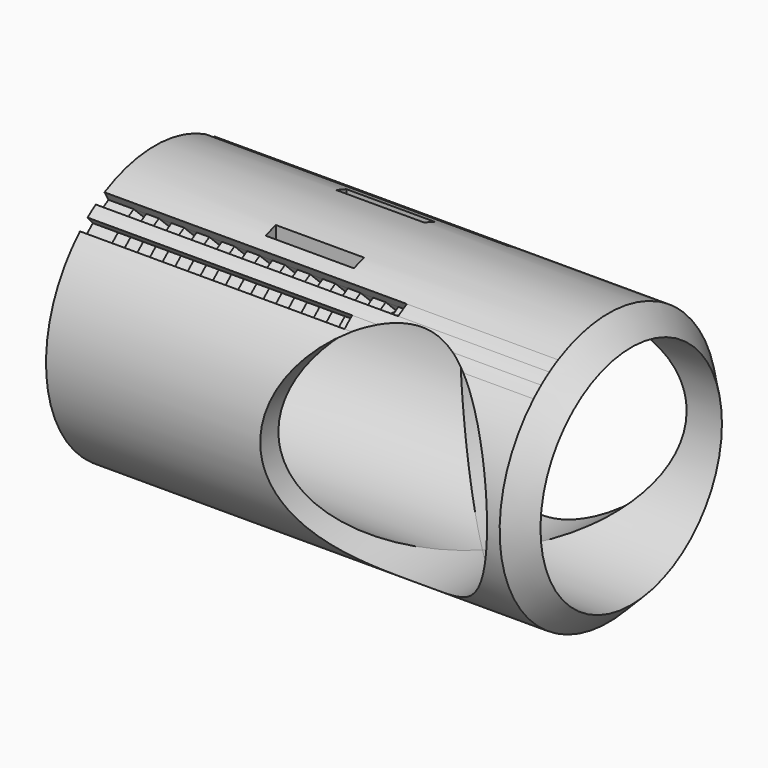
from build123d import *

# Parameters (mm, degrees)
F0_R      = 57.15
F1_DEPTH  = 241.3
F3_DEPTH  = 133.35
F4_DEPTH  = 152.4
F5_DEPTH  = 76.2
F10_ANGLE = 16.3
F11_W     = 44.45
F11_H     = 6.35
F12_DEPTH = 381


# Not quite as in the source:
# - a fillet or chamfer that OpenCascade refuses, or shapes differently, is made with other operations: its cross-section is extruded or revolved along the edge and cut away or added
# - a pattern or mirror of a feature is missing from the dataset's text; its kind, count and spacing are read off the source's solid


with BuildPart() as f1:
    # F0 (on Right) → F1 (new body)
    with BuildSketch(Plane.YZ):
        with BuildLine():
            ThreePointArc((-47.2070556813, 49.7464601143), (-27.0717243759, -63.0106192583), (68.58, 0))
            ThreePointArc((68.58, 0), (63.0106192583, 27.0717243759), (47.2070556813, 49.7464601143))
            Line((47.2070556813, 49.7464601143), (43.8845844861, 45.9035985298))
            Line((43.8845844861, 45.9035985298), (39.0810075056, 50.0566875238))
            Line((39.0810075056, 50.0566875238), (42.4034787008, 53.8995491082))
            ThreePointArc((42.4034787008, 53.8995491082), (39.8626621435, 55.8048794178), (37.2363602362, 57.5905363438))
            Line((37.2363602362, 57.5905363438), (34.6785672677, 53.2014481548))
            Line((34.6785672677, 53.2014481548), (29.1922070315, 56.3986893654))
            Line((29.1922070315, 56.3986893654), (31.75, 60.7877775544))
            ThreePointArc((31.75, 60.7877775544), (0, 68.58), (-31.75, 60.7877775544))
            Line((-31.75, 60.7877775544), (-29.1922070315, 56.3986893654))
            Line((-29.1922070315, 56.3986893654), (-34.6785672677, 53.2014481548))
            Line((-34.6785672677, 53.2014481548), (-37.2363602362, 57.5905363438))
            ThreePointArc((-37.2363602362, 57.5905363438), (-39.8626621435, 55.8048794178), (-42.4034787008, 53.8995491082))
            Line((-42.4034787008, 53.8995491082), (-39.0810075056, 50.0566875238))
            Line((-39.0810075056, 50.0566875238), (-43.8845844861, 45.9035985298))
            Line((-43.8845844861, 45.9035985298), (-47.2070556813, 49.7464601143))
        make_face()
        Circle(F0_R, mode=Mode.SUBTRACT)
        with BuildLine():
            ThreePointArc((-42.4034787008, 53.8995491082), (-44.853361135, 51.8786313899), (-47.2070556813, 49.7464601143))
            Line((-47.2070556813, 49.7464601143), (-43.8845844861, 45.9035985298))
            Line((-43.8845844861, 45.9035985298), (-39.0810075056, 50.0566875238))
            Line((-39.0810075056, 50.0566875238), (-42.4034787008, 53.8995491082))
        make_face()
        with BuildLine():
            ThreePointArc((-31.75, 60.7877775544), (-34.5302050747, 59.2526905507), (-37.2363602362, 57.5905363438))
            Line((-37.2363602362, 57.5905363438), (-34.6785672677, 53.2014481548))
            Line((-34.6785672677, 53.2014481548), (-29.1922070315, 56.3986893654))
            Line((-29.1922070315, 56.3986893654), (-31.75, 60.7877775544))
        make_face()
        with BuildLine():
            Line((34.6785672677, 53.2014481548), (37.2363602362, 57.5905363438))
            ThreePointArc((37.2363602362, 57.5905363438), (34.5302050747, 59.2526905507), (31.75, 60.7877775544))
            Line((31.75, 60.7877775544), (29.1922070315, 56.3986893654))
            Line((29.1922070315, 56.3986893654), (34.6785672677, 53.2014481548))
        make_face()
        with BuildLine():
            Line((43.8845844861, 45.9035985298), (47.2070556813, 49.7464601143))
            ThreePointArc((47.2070556813, 49.7464601143), (44.853361135, 51.8786313899), (42.4034787008, 53.8995491082))
            Line((42.4034787008, 53.8995491082), (39.0810075056, 50.0566875238))
            Line((39.0810075056, 50.0566875238), (43.8845844861, 45.9035985298))
        make_face()
    extrude(amount=F1_DEPTH)

    # F0 (on Right) → F3 (cut)
    with BuildSketch(Plane.YZ):
        with BuildLine():
            ThreePointArc((-42.4034787008, 53.8995491082), (-44.853361135, 51.8786313899), (-47.2070556813, 49.7464601143))
            Line((-47.2070556813, 49.7464601143), (-43.8845844861, 45.9035985298))
            Line((-43.8845844861, 45.9035985298), (-39.0810075056, 50.0566875238))
            Line((-39.0810075056, 50.0566875238), (-42.4034787008, 53.8995491082))
        make_face()
        with BuildLine():
            Line((43.8845844861, 45.9035985298), (47.2070556813, 49.7464601143))
            ThreePointArc((47.2070556813, 49.7464601143), (44.853361135, 51.8786313899), (42.4034787008, 53.8995491082))
            Line((42.4034787008, 53.8995491082), (39.0810075056, 50.0566875238))
            Line((39.0810075056, 50.0566875238), (43.8845844861, 45.9035985298))
        make_face()
    extrude(amount=F3_DEPTH, mode=Mode.SUBTRACT)

    # F0 (on Right) → F4 (cut)
    with BuildSketch(Plane.YZ):
        with BuildLine():
            ThreePointArc((-31.75, 60.7877775544), (-34.5302050747, 59.2526905507), (-37.2363602362, 57.5905363438))
            Line((-37.2363602362, 57.5905363438), (-34.6785672677, 53.2014481548))
            Line((-34.6785672677, 53.2014481548), (-29.1922070315, 56.3986893654))
            Line((-29.1922070315, 56.3986893654), (-31.75, 60.7877775544))
        make_face()
        with BuildLine():
            Line((34.6785672677, 53.2014481548), (37.2363602362, 57.5905363438))
            ThreePointArc((37.2363602362, 57.5905363438), (34.5302050747, 59.2526905507), (31.75, 60.7877775544))
            Line((31.75, 60.7877775544), (29.1922070315, 56.3986893654))
            Line((29.1922070315, 56.3986893654), (34.6785672677, 53.2014481548))
        make_face()
    extrude(amount=F4_DEPTH, mode=Mode.SUBTRACT)

    # F2 (on Front) → F5 (cut, symmetric)
    with BuildSketch(Plane.XZ):
        with BuildLine():
            ThreePointArc((107.95, 0), (165.1, -57.15), (222.25, 0))
            ThreePointArc((222.25, 0), (165.1, 57.15), (107.95, 0))
        make_face()
    extrude(amount=F5_DEPTH, both=True, mode=Mode.SUBTRACT)

    # F6: chamfer of 12.7 on 1 edges, made by hand

    # F6_s1 → F6_t2 (revolve, cut)
    with BuildSketch(Plane(origin=(0, 0, 0), x_dir=(1, 0, 0), z_dir=(0, 0.7253785377, -0.6883501849))):
        Polygon((228.6, -68.58), (241.3, -55.88), (241.3, -68.58), align=None)
    revolve(axis=Axis((241.3, 0, 0), (1, 0, 0)), mode=Mode.SUBTRACT)

    # F9 (on face) → F10 (revolve, cut)
    with BuildSketch(Plane(origin=(0, -2.7431801181, 1.5986206053), x_dir=(-1, 0, 0), z_dir=(0, 0.863993738, -0.5035025529))):
        Polygon((-152.2536198998, 57.0617373991), (-145.9036198998, 57.0617373991), (-139.7, 63.4264652058), (-146.05, 63.4264652058), align=None)
        Polygon((-139.5536198998, 57.0617373991), (-133.2036198998, 57.0617373991), (-127, 63.4264652058), (-133.35, 63.4264652058), align=None)
        Polygon((-126.8536198998, 57.0617373991), (-120.5036198998, 57.0617373991), (-114.3, 63.4264652058), (-120.65, 63.4264652058), align=None)
        Polygon((-114.1536198998, 57.0617373991), (-107.8036198998, 57.0617373991), (-101.6, 63.4264652058), (-107.95, 63.4264652058), align=None)
        Polygon((-101.4536198998, 57.0617373991), (-95.1036198998, 57.0617373991), (-88.9, 63.4264652058), (-95.25, 63.4264652058), align=None)
        Polygon((-88.7536198998, 57.0617373991), (-82.4036198998, 57.0617373991), (-76.2, 63.4264652058), (-82.55, 63.4264652058), align=None)
        Polygon((-76.0536198998, 57.0617373991), (-69.7036198998, 57.0617373991), (-63.5, 63.4264652058), (-69.85, 63.4264652058), align=None)
        Polygon((-63.3536198998, 57.0617373991), (-57.0036198998, 57.0617373991), (-50.8, 63.4264652058), (-57.15, 63.4264652058), align=None)
        Polygon((-50.6536198998, 57.0617373991), (-44.3036198998, 57.0617373991), (-38.1, 63.4264652058), (-44.45, 63.4264652058), align=None)
        Polygon((-37.9536198998, 57.0617373991), (-31.6036198998, 57.0617373991), (-25.4, 63.4264652058), (-31.75, 63.4264652058), align=None)
        Polygon((-25.2536198998, 57.0617373991), (-18.9036198998, 57.0617373991), (-12.7, 63.4264652058), (-19.05, 63.4264652058), align=None)
    f10 = revolve(axis=Axis((82.55, 0, 0), (-1, 0, 0)), revolution_arc=F10_ANGLE, mode=Mode.SUBTRACT)

    # F10_copies: F10 across plane
    add(f10.mirror(Plane(origin=(0, 0, 0), x_dir=(0, 0, -1), z_dir=(0, -1, 0))), mode=Mode.SUBTRACT)

    # F11 (on Top) → F12 (cut)
    with BuildSketch(Plane.XY):
        with Locations((98.425, -22.225)):
            Rectangle(F11_W, F11_H)
        with Locations((98.425, 22.225)):
            Rectangle(F11_W, F11_H)
    extrude(amount=F12_DEPTH, mode=Mode.SUBTRACT)


solid = f1.part
